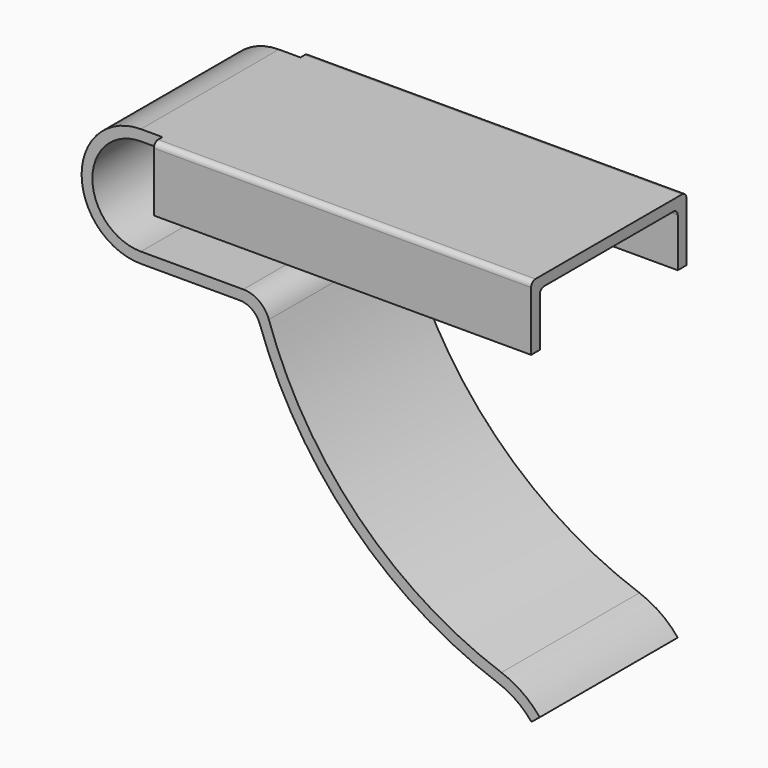
from build123d import *

# Parameters (mm, degrees)
F1_DEPTH = 16
F2_W     = 70
F2_H     = 2
F2_H_2   = 10
F3_DEPTH = 2
F4_R     = 1


with BuildPart() as f1:
    # F0 (on Front) → F1 (new body)
    with BuildSketch(Plane.XZ):
        with BuildLine():
            ThreePointArc((0, -9), (-9, 0), (0, 9))
            Line((0, 9), (74, 9))
            Line((74, 9), (74, 11))
            Line((74, 11), (0, 11))
            ThreePointArc((0, 11), (-11, 0), (0, -11))
            Line((0, -11), (18.2864816057, -11))
            ThreePointArc((18.2864816057, -11), (20.6021054823, -11.7384227646), (22.0627746665, -13.6810569689))
            ThreePointArc((22.0627746665, -13.6810569689), (39.0966080524, -40.824002055), (66.2209606463, -57.8874262169))
            ThreePointArc((66.2209606463, -57.8874262169), (69.6378774832, -59.6435957626), (72.4487811093, -62.2624262169))
            Line((72.4487811093, -62.2624262169), (74, -61))
            ThreePointArc((74, -61), (70.7875387131, -58.0070509094), (66.8824908995, -56))
            ThreePointArc((66.8824908995, -56), (40.2783781222, -39.1759850939), (23.7357366507, -12.396005494))
            ThreePointArc((23.7357366507, -12.396005494), (21.9137628138, -9.9367517594), (19, -9))
            Line((19, -9), (0, -9))
        make_face()
    extrude(amount=F1_DEPTH)

    # F2 (on face) → F3 (join)
    with BuildSketch(Plane.XZ.offset(16)):
        with Locations((39, 10)):
            Rectangle(F2_W, F2_H)
        with Locations((39, 4)):
            Rectangle(F2_W, F2_H_2)
    extrude(amount=F3_DEPTH)

    # F4
    f4_edges = [f1.edges().sort_by_distance(p)[0] for p in [
        (39, -18, 11),
        (39, -16, 9),
    ]]
    fillet(f4_edges, radius=F4_R)

    # F5: F1 across plane


with BuildPart() as f1_1:
    add(f1.part)
    add(f1.part.mirror(Plane.XZ))


solid = f1_1.part
